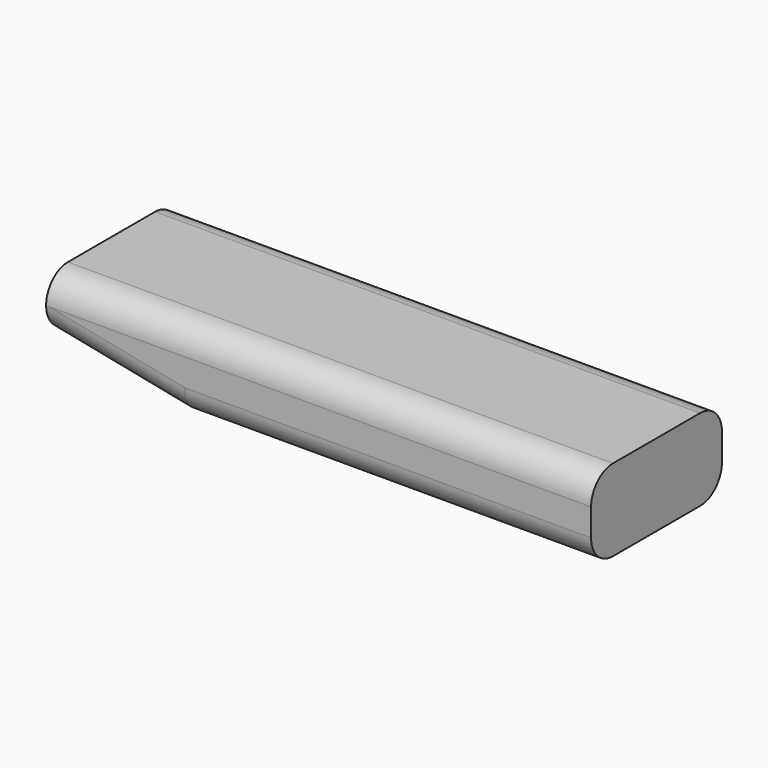
from build123d import *

# Parameters (mm, degrees)
F0_W        = 127
F0_H        = 38.1
F1_DEPTH    = 9.525
F2_R        = 15.875
F3_DEPTH    = 12.7
F5_DEPTH    = 4.7625
F7_DEPTH    = 38.101
F8_T1_DEPTH = 158.75
F8_T3_DEPTH = 95.8787739113
F8_T5_DEPTH = 95.8787739113


# Not quite as in the source:
# - a fillet or chamfer that OpenCascade refuses, or shapes differently, is made with other operations: its cross-section is extruded or revolved along the edge and cut away or added


with BuildPart() as f1:
    # F0 (on Top) → F1 (new body, symmetric)
    with BuildSketch(Plane.XY):
        Rectangle(F0_W, F0_H)
    extrude(amount=F1_DEPTH, both=True)

    # F2 (on face) → F3 (cut)
    with BuildSketch(Plane(origin=(0, 0, -9.525), x_dir=(1, 0, 0), z_dir=(0, 0, -1))):
        with Locations((-44.45, 0)):
            Circle(F2_R)
    extrude(amount=-F3_DEPTH, mode=Mode.SUBTRACT)

    # F4 (on face) → F5 (cut)
    with BuildSketch(Plane(origin=(0, 0, -9.525), x_dir=(1, 0, 0), z_dir=(0, 0, -1))):
        with BuildLine():
            ThreePointArc((-31.2964285714, -8.8881484952), (-17.4248511928, -11.7579152671), (-9.525, 0))
            ThreePointArc((-9.525, 0), (-17.4248511928, 11.7579152671), (-31.2964285714, 8.8881484952))
            ThreePointArc((-31.2964285714, 8.8881484952), (-29.2705966615, 4.6477240974), (-28.575, 0))
            ThreePointArc((-28.575, 0), (-29.2705966615, -4.6477240974), (-31.2964285714, -8.8881484952))
        make_face()
    extrude(amount=-F5_DEPTH, mode=Mode.SUBTRACT)

    # F6 (on face) → F7 (cut, through all)
    with BuildSketch(Plane(origin=(0, 19.05, 0), x_dir=(-1, 0, 0), z_dir=(0, 1, 0))):
        Polygon((31.75, -9.525), (63.5, -9.525), (63.5, -3.175), align=None)
    extrude(amount=-F7_DEPTH, mode=Mode.SUBTRACT)

    # F8: fillet of radius 6.35 on 6 edges, made by hand

    # F8_s2 → F8_t1 (cut)
    with BuildSketch(Plane.YZ.offset(-79.375)):
        with BuildLine():
            ThreePointArc((-12.7, 9.525), (-17.1901280605, 7.6651280605), (-19.05, 3.175))
            Line((-19.05, 3.175), (-19.05, 9.525))
            Line((-19.05, 9.525), (-12.7, 9.525))
        make_face()
        with BuildLine():
            ThreePointArc((19.05, 3.175), (17.1901280605, 7.6651280605), (12.7, 9.525))
            Line((12.7, 9.525), (19.05, 9.525))
            Line((19.05, 9.525), (19.05, 3.175))
        make_face()
        with BuildLine():
            ThreePointArc((-12.7, -9.525), (-17.1901280605, -7.6651280605), (-19.05, -3.175))
            Line((-19.05, -3.175), (-19.05, -9.525))
            Line((-19.05, -9.525), (-12.7, -9.525))
        make_face()
        with BuildLine():
            ThreePointArc((19.05, -3.175), (17.1901280605, -7.6651280605), (12.7, -9.525))
            Line((12.7, -9.525), (19.05, -9.525))
            Line((19.05, -9.525), (19.05, -3.175))
        make_face()
    extrude(amount=F8_T1_DEPTH, mode=Mode.SUBTRACT)

    # F8_s4 → F8_t3 (cut)
    with BuildSketch(Plane(origin=(-76.0138336112, 0, 15.2027667222), x_dir=(0, 1, 0), z_dir=(0.9805806757, 0, -0.1961161351))):
        with BuildLine():
            ThreePointArc((19.05, -9.2167182266), (17.1901280605, -13.7068462871), (12.7, -15.5667182266))
            Line((12.7, -15.5667182266), (19.05, -15.5667182266))
            Line((19.05, -15.5667182266), (19.05, -9.2167182266))
        make_face()
    extrude(amount=F8_T3_DEPTH, mode=Mode.SUBTRACT)

    # F8_s6 → F8_t5 (cut)
    with BuildSketch(Plane(origin=(18.0030392952, 0, -3.600607859), x_dir=(0, 1, 0), z_dir=(-0.9805806757, 0, 0.1961161351))):
        with BuildLine():
            ThreePointArc((-12.7, 15.5667182266), (-17.1901280605, 13.7068462871), (-19.05, 9.2167182266))
            Line((-19.05, 9.2167182266), (-19.05, 15.5667182266))
            Line((-19.05, 15.5667182266), (-12.7, 15.5667182266))
        make_face()
    extrude(amount=F8_T5_DEPTH, mode=Mode.SUBTRACT)


solid = f1.part
